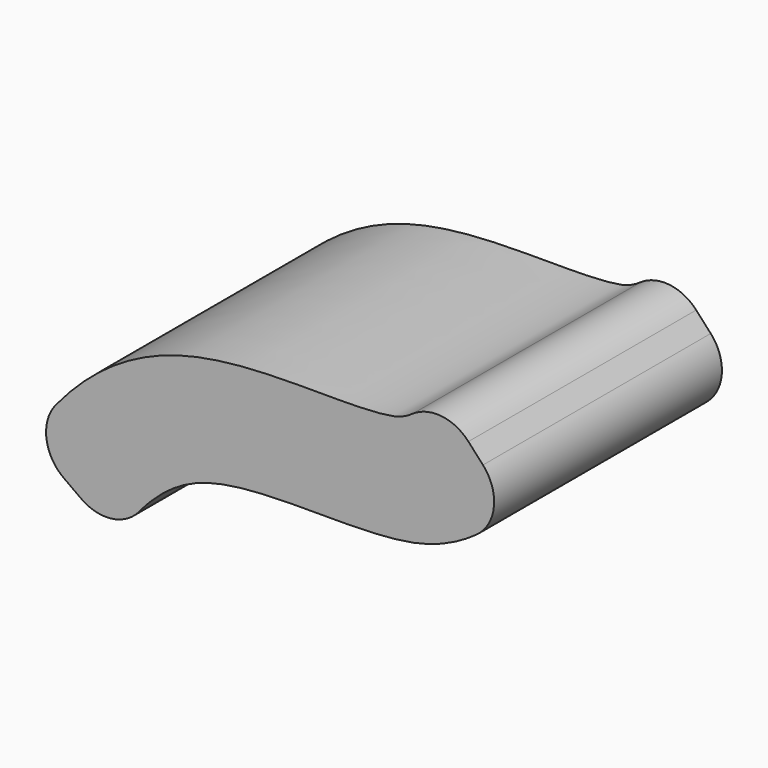
from build123d import *

# Parameters (mm, degrees)
F1_DEPTH = 50.8
F2_R     = 7.62


# Not quite as in the source:
# - the dataset's text gives a spline's control points without its knots; the knots are read off the source's solid


with BuildPart() as f1:
    # F0 (on Front) → F1 (new body)
    with BuildSketch(Plane.XZ):
        with BuildLine():
            Line((-66.5414150367, 7.9755592532), (-51.0662905872, -3.1340322457))
            add(Edge.make_bspline(
                [(-51.0662905872, -3.1340322457), (-46.9080086103, 2.6582537348), (-37.2164193187, 16.158169588), (3.9661427847, 9.376928998), (15.1752961857, 19.6334986968), (19.9103225023, 23.9661298692)],
                knots=[0, 0, 0, 0, 0.302673171, 0.7054317335, 1, 1, 1, 1], degree=3))
            Line((19.9103225023, 23.9661298692), (7.0503695481, 38.0204569615))
            add(Edge.make_bspline(
                [(-66.5414150367, 7.9755592532), (-65.6827574204, 9.1716278461), (-64.2376881581, 11.1925403484), (-61.8537311601, 14.230245381), (-59.7849919212, 16.6397090343), (-57.3812599932, 19.1267056888), (-54.5913152498, 21.616929755), (-51.9156052216, 23.6141415002), (-49.5636524979, 25.1087524342), (-47.6977784369, 26.1638231657), (-45.7360020225, 27.1394154139), (-43.6849425957, 28.0238468654), (-41.9133563994, 28.6753866943), (-40.4544972877, 29.1442267499), (-39.3706343495, 29.4604482596), (-38.3024046597, 29.7433243724), (-36.8966327798, 30.0805873366), (-34.4850412565, 30.5755105454), (-31.1673262141, 31.0605685349), (-27.3563371493, 31.4025851529), (-23.6940833425, 31.582346389), (-20.1745271825, 31.65755623), (-15.6846174083, 31.6781564731), (-11.5360581226, 31.6568797923), (-7.8877151981, 31.7097261242), (-5.4640436851, 31.8039348118), (-3.7669566424, 31.9346358754), (-2.6503542293, 32.0634185934), (-2.0645638727, 32.1496749584), (-1.6701914585, 32.2182935913), (-1.4140790271, 32.2680724783), (-1.1968720881, 32.3150339788), (-0.9185781733, 32.3814206056), (-0.6019359075, 32.4682882445), (-0.1412938907, 32.6163591904), (0.3743523739, 32.8201499972), (0.9825969287, 33.1187793404), (1.6485537837, 33.510239909), (2.6765705542, 34.2100049696), (4.3015951848, 35.5125797753), (6.0457156922, 37.1011812653), (7.0503695481, 38.0204569615)],
                knots=[0, 0, 0, 0, 0.0625, 0.09375, 0.125, 0.15625, 0.1875, 0.21875, 0.234375, 0.25, 0.265625, 0.28125, 0.296875, 0.3046875, 0.3125, 0.3203125, 0.328125, 0.34375, 0.375, 0.40625, 0.4375, 0.46875, 0.5, 0.5625, 0.59375, 0.625, 0.65625, 0.671875, 0.6875, 0.6953125, 0.703125, 0.7109375, 0.71875, 0.734375, 0.75, 0.78125, 0.8125, 0.84375, 0.875, 0.9375, 1, 1, 1, 1], degree=3))
        make_face()
    extrude(amount=F1_DEPTH)

    # F2
    f2_edges = [f1.edges().sort_by_distance(p)[0] for p in [
        (7.05037, -25.4, 38.020457),
        (19.910323, -25.4, 23.96613),
        (-66.541415, -25.4, 7.975559),
        (-51.066291, -25.4, -3.134032),
    ]]
    fillet(f2_edges, radius=F2_R)


solid = f1.part
